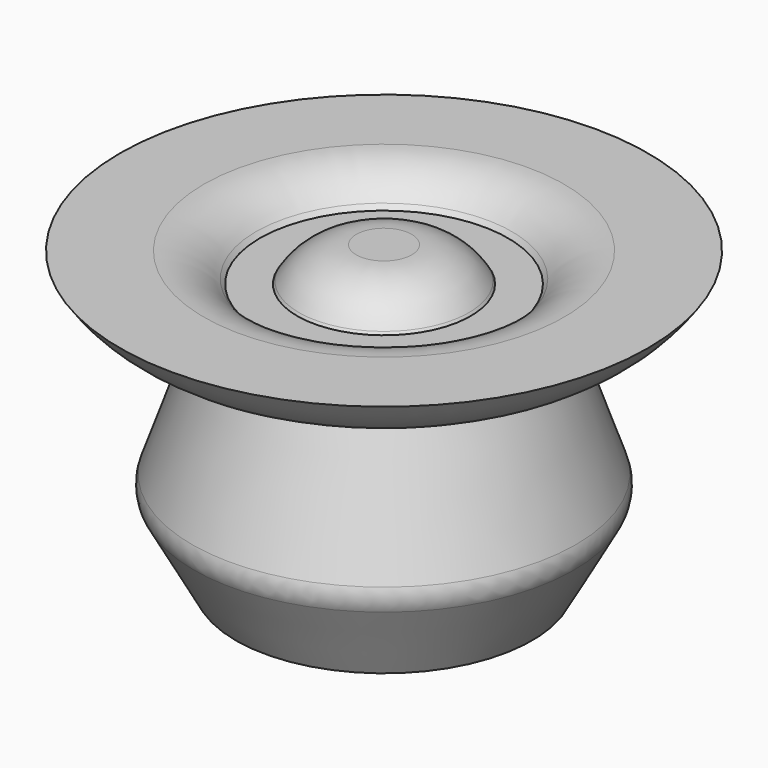
from build123d import *

# Parameters (mm, degrees)
F3_R = 2.1064176113
F4_R = 5


# Not quite as in the source:
# - a fillet or chamfer that OpenCascade refuses, or shapes differently, is made with other operations: its cross-section is extruded or revolved along the edge and cut away or added


with BuildPart() as f1:
    # F0 (on Front) → F1 (revolve)
    with BuildSketch(Plane.XZ):
        Polygon((-10.9814703465, 0), (0, 0), (0, 22.2597364336), (-4.8476760276, 22.2597364336), (-6.4305909909, 19.6906365962), (-9.2006912455, 19.6906365962), (-10.9814703465, 21.8640081584), (-19.5646515468, 21.8640081584), (-19.5646515468, 19.6906365962), (-10.9814703465, 16.7195349932), (-14.5430285484, 6.4305905253), align=None)
    revolve(axis=Axis((0, 0, 11.1298682168), (0, 0, -1)))

    # F2: fillet of radius 10.1048761085 on 1 edges, made by hand

    # F2_s1 → F2_t2 (revolve, cut)
    with BuildSketch(Plane.XZ):
        with BuildLine():
            ThreePointArc((-19.5646515468, 21.8640081584), (-17.3375812271, 19.4776240652), (-14.4659586897, 17.9257042049))
            Line((-14.4659586897, 17.9257042049), (-19.5646515468, 19.6906365962))
            Line((-19.5646515468, 19.6906365962), (-19.5646515468, 21.8640081584))
        make_face()
    revolve(axis=Axis((0, 0, 19.6906365962), (0, 0, -1)), mode=Mode.SUBTRACT)

    # F3
    f3_edges = [f1.edges().sort_by_distance(p)[0] for p in [
        (14.543029, 0, 6.430591),
    ]]
    fillet(f3_edges, radius=F3_R)

    # F4
    f4_edges = [f1.edges().sort_by_distance(p)[0] for p in [
        (10.98147, 0, 21.864008),
        (4.847676, 0, 22.259736),
    ]]
    fillet(f4_edges, radius=F4_R)


solid = f1.part
